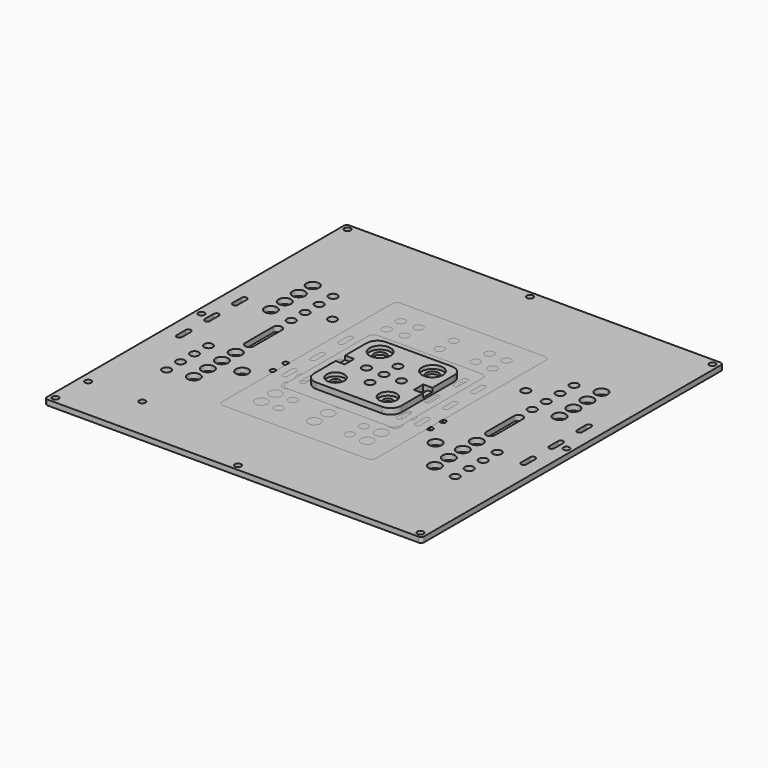
from build123d import *

# Parameters (mm, degrees)
F0_R      = 1.8
F0_R_2    = 2.5
F0_R_3    = 3.6
F0_R_4    = 1.57
F0_R_5    = 1.75
F1_DEPTH  = 3
F2_R      = 3.55
F2_R_2    = 2.55
F3_DEPTH  = 3
F5_R      = 5.05
F5_R_2    = 2.51
F5_R_3    = 6
F6_DEPTH  = 6.35
F5_R_4    = 3.57
F5_R_5    = 2.5
F7_DEPTH  = 4.35
F5_W      = 2.75
F5_H      = 6.7
F8_DEPTH  = 4.17
F9_R      = 3.6
F9_R_2    = 2.5
F10_DEPTH = 3


with BuildPart() as f1:
    # F0 (on Top) → F1 (new body)
    with BuildSketch(Plane.XY):
        with BuildLine():
            Line((106.25, 108), (-106.25, 108))
            ThreePointArc((-106.25, 108), (-107.4874368671, 107.4874368671), (-108, 106.25))
            Line((-108, 106.25), (-108, -106.25))
            ThreePointArc((-108, -106.25), (-107.4874368671, -107.4874368671), (-106.25, -108))
            Line((-106.25, -108), (106.25, -108))
            ThreePointArc((106.25, -108), (107.4874368671, -107.4874368671), (108, -106.25))
            Line((108, -106.25), (108, 106.25))
            ThreePointArc((108, 106.25), (107.4874368671, 107.4874368671), (106.25, 108))
        make_face()
        with Locations((-104.5, -104.5)):
            Circle(F0_R, mode=Mode.SUBTRACT)
        with Locations((-103, -83)):
            Circle(F0_R, mode=Mode.SUBTRACT)
        with Locations((-72, -83)):
            Circle(F0_R, mode=Mode.SUBTRACT)
        with Locations((-82.65, -52.3)):
            Circle(F0_R_2, mode=Mode.SUBTRACT)
        with Locations((-82.65, -42.3)):
            Circle(F0_R_2, mode=Mode.SUBTRACT)
        with Locations((-82.65, -32.3)):
            Circle(F0_R_2, mode=Mode.SUBTRACT)
        with Locations((-69, -49.85)):
            Circle(F0_R_3, mode=Mode.SUBTRACT)
        with Locations((-69, -39.85)):
            Circle(F0_R_3, mode=Mode.SUBTRACT)
        with Locations((-69, -29.85)):
            Circle(F0_R_3, mode=Mode.SUBTRACT)
        with Locations((-55.35, -32.3)):
            Circle(F0_R_3, mode=Mode.SUBTRACT)
        with BuildLine():
            Line((-100.12, -23.25), (-100.12, -16.75))
            ThreePointArc((-100.12, -16.75), (-98.62, -15.25), (-97.12, -16.75))
            Line((-97.12, -16.75), (-97.12, -23.25))
            ThreePointArc((-97.12, -23.25), (-98.62, -24.75), (-100.12, -23.25))
        make_face(mode=Mode.SUBTRACT)
        with Locations((-82.65, -22.3)):
            Circle(F0_R_2, mode=Mode.SUBTRACT)
        with Locations((-69, -19.85)):
            Circle(F0_R_3, mode=Mode.SUBTRACT)
        with Locations((-20.325, -30.32)):
            Circle(F0_R_2, mode=Mode.SUBTRACT)
        with Locations((-45, -23.12)):
            Circle(F0_R_4, mode=Mode.SUBTRACT)
        with Locations((-45, -14)):
            Circle(F0_R_4, mode=Mode.SUBTRACT)
        with Locations((-28, -12.64)):
            Circle(F0_R_5, mode=Mode.SUBTRACT)
        with Locations((-28, -2.5)):
            Circle(F0_R_5, mode=Mode.SUBTRACT)
        with Locations((-10.16, -20.32)):
            Circle(F0_R_2, mode=Mode.SUBTRACT)
        with Locations((-15.17, -12.64)):
            Circle(F0_R_5, mode=Mode.SUBTRACT)
        with Locations((-15.17, -2.5)):
            Circle(F0_R_5, mode=Mode.SUBTRACT)
        with Locations((0, -104.5)):
            Circle(F0_R, mode=Mode.SUBTRACT)
        with Locations((104.5, -104.5)):
            Circle(F0_R, mode=Mode.SUBTRACT)
        with Locations((20.325, -30.32)):
            Circle(F0_R_2, mode=Mode.SUBTRACT)
        with Locations((10.16, -20.32)):
            Circle(F0_R_2, mode=Mode.SUBTRACT)
        with Locations((0, -10)):
            Circle(F0_R_2, mode=Mode.SUBTRACT)
        with Locations((45, -23.12)):
            Circle(F0_R_4, mode=Mode.SUBTRACT)
        with Locations((45, -14)):
            Circle(F0_R_4, mode=Mode.SUBTRACT)
        with Locations((69, -49.85)):
            Circle(F0_R_3, mode=Mode.SUBTRACT)
        with Locations((55.35, -32.3)):
            Circle(F0_R_3, mode=Mode.SUBTRACT)
        with Locations((69, -39.85)):
            Circle(F0_R_3, mode=Mode.SUBTRACT)
        with Locations((69, -29.85)):
            Circle(F0_R_3, mode=Mode.SUBTRACT)
        with Locations((82.65, -52.3)):
            Circle(F0_R_2, mode=Mode.SUBTRACT)
        with Locations((82.65, -42.3)):
            Circle(F0_R_2, mode=Mode.SUBTRACT)
        with Locations((82.65, -32.3)):
            Circle(F0_R_2, mode=Mode.SUBTRACT)
        with Locations((69, -19.85)):
            Circle(F0_R_3, mode=Mode.SUBTRACT)
        with Locations((82.65, -22.3)):
            Circle(F0_R_2, mode=Mode.SUBTRACT)
        with BuildLine():
            Line((97.12, -23.25), (97.12, -16.75))
            ThreePointArc((97.12, -16.75), (98.62, -15.25), (100.12, -16.75))
            Line((100.12, -16.75), (100.12, -23.25))
            ThreePointArc((100.12, -23.25), (98.62, -24.75), (97.12, -23.25))
        make_face(mode=Mode.SUBTRACT)
        with Locations((-104.5, 0)):
            Circle(F0_R, mode=Mode.SUBTRACT)
        with BuildLine():
            ThreePointArc((-100.12, 3.25), (-98.62, 4.75), (-97.12, 3.25))
            Line((-97.12, 3.25), (-97.12, -3.25))
            ThreePointArc((-97.12, -3.25), (-98.62, -4.75), (-100.12, -3.25))
            Line((-100.12, -3.25), (-100.12, 3.25))
        make_face(mode=Mode.SUBTRACT)
        with BuildLine():
            ThreePointArc((-100.12, 23.25), (-98.62, 24.75), (-97.12, 23.25))
            Line((-97.12, 23.25), (-97.12, 16.75))
            ThreePointArc((-97.12, 16.75), (-98.62, 15.25), (-100.12, 16.75))
            Line((-100.12, 16.75), (-100.12, 23.25))
        make_face(mode=Mode.SUBTRACT)
        with Locations((-82.65, 22.3)):
            Circle(F0_R_3, mode=Mode.SUBTRACT)
        with BuildLine():
            Line((-66.5, 10), (-66.5, -10))
            ThreePointArc((-66.5, -10), (-69, -12.5), (-71.5, -10))
            Line((-71.5, -10), (-71.5, 10))
            ThreePointArc((-71.5, 10), (-69, 12.5), (-66.5, 10))
        make_face(mode=Mode.SUBTRACT)
        with Locations((-69, 19.85)):
            Circle(F0_R_2, mode=Mode.SUBTRACT)
        with Locations((-82.65, 32.3)):
            Circle(F0_R_3, mode=Mode.SUBTRACT)
        with Locations((-82.65, 42.3)):
            Circle(F0_R_3, mode=Mode.SUBTRACT)
        with Locations((-82.65, 52.3)):
            Circle(F0_R_3, mode=Mode.SUBTRACT)
        with Locations((-69, 29.85)):
            Circle(F0_R_2, mode=Mode.SUBTRACT)
        with Locations((-69, 39.85)):
            Circle(F0_R_2, mode=Mode.SUBTRACT)
        with Locations((-55.35, 32.3)):
            Circle(F0_R_2, mode=Mode.SUBTRACT)
        with Locations((-69, 49.85)):
            Circle(F0_R_2, mode=Mode.SUBTRACT)
        with Locations((-10.16, 20.32)):
            Circle(F0_R_2, mode=Mode.SUBTRACT)
        with Locations((-20.325, 30.32)):
            Circle(F0_R_2, mode=Mode.SUBTRACT)
        with Locations((-104.5, 104.5)):
            Circle(F0_R, mode=Mode.SUBTRACT)
        Circle(F0_R, mode=Mode.SUBTRACT)
        with Locations((0, 10)):
            Circle(F0_R_2, mode=Mode.SUBTRACT)
        with Locations((10.16, 20.32)):
            Circle(F0_R_2, mode=Mode.SUBTRACT)
        with Locations((20.325, 30.32)):
            Circle(F0_R_2, mode=Mode.SUBTRACT)
        with BuildLine():
            ThreePointArc((71.5, -10), (69, -12.5), (66.5, -10))
            Line((66.5, -10), (66.5, 10))
            ThreePointArc((66.5, 10), (69, 12.5), (71.5, 10))
            Line((71.5, 10), (71.5, -10))
        make_face(mode=Mode.SUBTRACT)
        with Locations((69, 19.85)):
            Circle(F0_R_2, mode=Mode.SUBTRACT)
        with BuildLine():
            ThreePointArc((100.12, -3.25), (98.62, -4.75), (97.12, -3.25))
            Line((97.12, -3.25), (97.12, 3.25))
            ThreePointArc((97.12, 3.25), (98.62, 4.75), (100.12, 3.25))
            Line((100.12, 3.25), (100.12, -3.25))
        make_face(mode=Mode.SUBTRACT)
        with Locations((104.5, 0)):
            Circle(F0_R, mode=Mode.SUBTRACT)
        with Locations((82.65, 22.3)):
            Circle(F0_R_3, mode=Mode.SUBTRACT)
        with BuildLine():
            Line((97.12, 16.75), (97.12, 23.25))
            ThreePointArc((97.12, 23.25), (98.62, 24.75), (100.12, 23.25))
            Line((100.12, 23.25), (100.12, 16.75))
            ThreePointArc((100.12, 16.75), (98.62, 15.25), (97.12, 16.75))
        make_face(mode=Mode.SUBTRACT)
        with Locations((55.35, 32.3)):
            Circle(F0_R_2, mode=Mode.SUBTRACT)
        with Locations((69, 29.85)):
            Circle(F0_R_2, mode=Mode.SUBTRACT)
        with Locations((69, 39.85)):
            Circle(F0_R_2, mode=Mode.SUBTRACT)
        with Locations((69, 49.85)):
            Circle(F0_R_2, mode=Mode.SUBTRACT)
        with Locations((82.65, 32.3)):
            Circle(F0_R_3, mode=Mode.SUBTRACT)
        with Locations((82.65, 42.3)):
            Circle(F0_R_3, mode=Mode.SUBTRACT)
        with Locations((82.65, 52.3)):
            Circle(F0_R_3, mode=Mode.SUBTRACT)
        with Locations((0, 104.5)):
            Circle(F0_R, mode=Mode.SUBTRACT)
        with Locations((104.5, 104.5)):
            Circle(F0_R, mode=Mode.SUBTRACT)
    extrude(amount=F1_DEPTH)


with BuildPart() as f3:
    # F2 (on Top) → F3 (new body)
    with BuildSketch(Plane.XY):
        with BuildLine():
            Line((41, 63.5), (-41, 63.5))
            ThreePointArc((-41, 63.5), (-43.1213203436, 62.6213203436), (-44, 60.5))
            Line((-44, 60.5), (-44, -60.5))
            ThreePointArc((-44, -60.5), (-43.1213203436, -62.6213203436), (-41, -63.5))
            Line((-41, -63.5), (41, -63.5))
            ThreePointArc((41, -63.5), (43.1213203436, -62.6213203436), (44, -60.5))
            Line((44, -60.5), (44, 60.5))
            ThreePointArc((44, 60.5), (43.1213203436, 62.6213203436), (41, 63.5))
        make_face()
        with Locations((-30.32, -49.85)):
            Circle(F2_R, mode=Mode.SUBTRACT)
        with Locations((-30.32, -39.85)):
            Circle(F2_R, mode=Mode.SUBTRACT)
        with Locations((-20.32, -49.85)):
            Circle(F2_R_2, mode=Mode.SUBTRACT)
        with Locations((-20.32, -39.85)):
            Circle(F2_R_2, mode=Mode.SUBTRACT)
        with BuildLine():
            ThreePointArc((-39.5, -16.75), (-38, -15.25), (-36.5, -16.75))
            Line((-36.5, -16.75), (-36.5, -23.25))
            ThreePointArc((-36.5, -23.25), (-38, -24.75), (-39.5, -23.25))
            Line((-39.5, -23.25), (-39.5, -16.75))
        make_face(mode=Mode.SUBTRACT)
        with Locations((-30.32, -29.85)):
            Circle(F2_R, mode=Mode.SUBTRACT)
        with Locations((-30.32, -19.85)):
            Circle(F2_R, mode=Mode.SUBTRACT)
        with Locations((-20.32, -29.85)):
            Circle(F2_R_2, mode=Mode.SUBTRACT)
        with Locations((-20.32, -19.85)):
            Circle(F2_R_2, mode=Mode.SUBTRACT)
        with Locations((-10, -30.32)):
            Circle(F2_R_2, mode=Mode.SUBTRACT)
        with Locations((-10, -20.32)):
            Circle(F2_R_2, mode=Mode.SUBTRACT)
        with Locations((-20.32, -9.85)):
            Circle(F2_R_2, mode=Mode.SUBTRACT)
        with Locations((-14.825, -14.825)):
            Circle(F2_R_2, mode=Mode.SUBTRACT)
        with Locations((0, -49.85)):
            Circle(F2_R, mode=Mode.SUBTRACT)
        with Locations((20.32, -49.85)):
            Circle(F2_R_2, mode=Mode.SUBTRACT)
        with Locations((0, -39.85)):
            Circle(F2_R, mode=Mode.SUBTRACT)
        with Locations((20.32, -39.85)):
            Circle(F2_R_2, mode=Mode.SUBTRACT)
        with Locations((30.32, -49.85)):
            Circle(F2_R, mode=Mode.SUBTRACT)
        with Locations((30.32, -39.85)):
            Circle(F2_R, mode=Mode.SUBTRACT)
        with Locations((0, -29.85)):
            Circle(F2_R, mode=Mode.SUBTRACT)
        with Locations((10, -30.32)):
            Circle(F2_R_2, mode=Mode.SUBTRACT)
        with Locations((0, -19.85)):
            Circle(F2_R, mode=Mode.SUBTRACT)
        with Locations((10, -20.32)):
            Circle(F2_R_2, mode=Mode.SUBTRACT)
        with Locations((20.32, -29.85)):
            Circle(F2_R_2, mode=Mode.SUBTRACT)
        with Locations((20.32, -19.85)):
            Circle(F2_R_2, mode=Mode.SUBTRACT)
        with Locations((0, -10)):
            Circle(F2_R_2, mode=Mode.SUBTRACT)
        with Locations((14.825, -14.825)):
            Circle(F2_R_2, mode=Mode.SUBTRACT)
        with Locations((20.32, -9.85)):
            Circle(F2_R_2, mode=Mode.SUBTRACT)
        with Locations((30.32, -29.85)):
            Circle(F2_R, mode=Mode.SUBTRACT)
        with Locations((30.32, -19.85)):
            Circle(F2_R, mode=Mode.SUBTRACT)
        with BuildLine():
            Line((36.5, -23.25), (36.5, -16.75))
            ThreePointArc((36.5, -16.75), (38, -15.25), (39.5, -16.75))
            Line((39.5, -16.75), (39.5, -23.25))
            ThreePointArc((39.5, -23.25), (38, -24.75), (36.5, -23.25))
        make_face(mode=Mode.SUBTRACT)
        with BuildLine():
            Line((-39.5, -3.25), (-39.5, 3.25))
            ThreePointArc((-39.5, 3.25), (-38, 4.75), (-36.5, 3.25))
            Line((-36.5, 3.25), (-36.5, -3.25))
            ThreePointArc((-36.5, -3.25), (-38, -4.75), (-39.5, -3.25))
        make_face(mode=Mode.SUBTRACT)
        with BuildLine():
            Line((-27.82, 10), (-27.82, -10))
            ThreePointArc((-27.82, -10), (-30.32, -12.5), (-32.82, -10))
            Line((-32.82, -10), (-32.82, 10))
            ThreePointArc((-32.82, 10), (-30.32, 12.5), (-27.82, 10))
        make_face(mode=Mode.SUBTRACT)
        with BuildLine():
            Line((-36.5, 23.25), (-36.5, 16.75))
            ThreePointArc((-36.5, 16.75), (-38, 15.25), (-39.5, 16.75))
            Line((-39.5, 16.75), (-39.5, 23.25))
            ThreePointArc((-39.5, 23.25), (-38, 24.75), (-36.5, 23.25))
        make_face(mode=Mode.SUBTRACT)
        with Locations((-30.32, 19.85)):
            Circle(F2_R_2, mode=Mode.SUBTRACT)
        with Locations((-30.32, 29.85)):
            Circle(F2_R_2, mode=Mode.SUBTRACT)
        with Locations((-20.32, 0.15)):
            Circle(F2_R_2, mode=Mode.SUBTRACT)
        with Locations((-20.32, 10.15)):
            Circle(F2_R_2, mode=Mode.SUBTRACT)
        with Locations((-14.825, 14.825)):
            Circle(F2_R_2, mode=Mode.SUBTRACT)
        with Locations((-10, 0)):
            Circle(F2_R_2, mode=Mode.SUBTRACT)
        with Locations((-20.32, 20.15)):
            Circle(F2_R_2, mode=Mode.SUBTRACT)
        with Locations((-20.32, 30.15)):
            Circle(F2_R_2, mode=Mode.SUBTRACT)
        with Locations((-10, 20.32)):
            Circle(F2_R_2, mode=Mode.SUBTRACT)
        with Locations((-10, 30.32)):
            Circle(F2_R_2, mode=Mode.SUBTRACT)
        with Locations((-30.32, 39.85)):
            Circle(F2_R_2, mode=Mode.SUBTRACT)
        with Locations((-30.32, 49.85)):
            Circle(F2_R_2, mode=Mode.SUBTRACT)
        with Locations((-20.32, 40.15)):
            Circle(F2_R_2, mode=Mode.SUBTRACT)
        with Locations((-20.32, 50.15)):
            Circle(F2_R_2, mode=Mode.SUBTRACT)
        Circle(F2_R_2, mode=Mode.SUBTRACT)
        with Locations((10, 0)):
            Circle(F2_R_2, mode=Mode.SUBTRACT)
        with Locations((0, 10)):
            Circle(F2_R_2, mode=Mode.SUBTRACT)
        with Locations((20.32, 0.15)):
            Circle(F2_R_2, mode=Mode.SUBTRACT)
        with Locations((14.825, 14.825)):
            Circle(F2_R_2, mode=Mode.SUBTRACT)
        with Locations((20.32, 10.15)):
            Circle(F2_R_2, mode=Mode.SUBTRACT)
        with Locations((0, 19.85)):
            Circle(F2_R_2, mode=Mode.SUBTRACT)
        with Locations((10, 20.32)):
            Circle(F2_R_2, mode=Mode.SUBTRACT)
        with Locations((0, 29.85)):
            Circle(F2_R_2, mode=Mode.SUBTRACT)
        with Locations((10, 30.32)):
            Circle(F2_R_2, mode=Mode.SUBTRACT)
        with Locations((20.32, 20.15)):
            Circle(F2_R_2, mode=Mode.SUBTRACT)
        with Locations((20.32, 30.15)):
            Circle(F2_R_2, mode=Mode.SUBTRACT)
        with BuildLine():
            Line((32.82, 10), (32.82, -10))
            ThreePointArc((32.82, -10), (30.32, -12.5), (27.82, -10))
            Line((27.82, -10), (27.82, 10))
            ThreePointArc((27.82, 10), (30.32, 12.5), (32.82, 10))
        make_face(mode=Mode.SUBTRACT)
        with BuildLine():
            ThreePointArc((36.5, 3.25), (38, 4.75), (39.5, 3.25))
            Line((39.5, 3.25), (39.5, -3.25))
            ThreePointArc((39.5, -3.25), (38, -4.75), (36.5, -3.25))
            Line((36.5, -3.25), (36.5, 3.25))
        make_face(mode=Mode.SUBTRACT)
        with Locations((30.32, 19.85)):
            Circle(F2_R_2, mode=Mode.SUBTRACT)
        with Locations((30.32, 29.85)):
            Circle(F2_R_2, mode=Mode.SUBTRACT)
        with BuildLine():
            ThreePointArc((36.5, 23.25), (38, 24.75), (39.5, 23.25))
            Line((39.5, 23.25), (39.5, 16.75))
            ThreePointArc((39.5, 16.75), (38, 15.25), (36.5, 16.75))
            Line((36.5, 16.75), (36.5, 23.25))
        make_face(mode=Mode.SUBTRACT)
        with Locations((0, 39.85)):
            Circle(F2_R_2, mode=Mode.SUBTRACT)
        with Locations((20.32, 40.15)):
            Circle(F2_R_2, mode=Mode.SUBTRACT)
        with Locations((0, 49.85)):
            Circle(F2_R_2, mode=Mode.SUBTRACT)
        with Locations((20.32, 50.15)):
            Circle(F2_R_2, mode=Mode.SUBTRACT)
        with Locations((30.32, 39.85)):
            Circle(F2_R_2, mode=Mode.SUBTRACT)
        with Locations((30.32, 49.85)):
            Circle(F2_R_2, mode=Mode.SUBTRACT)
    extrude(amount=F3_DEPTH)


with BuildPart() as f6:
    # F5 (on Top) → F6 (new body)
    with BuildSketch(Plane.XY):
        with BuildLine():
            Line((-18.83, -25), (18.83, -25))
            ThreePointArc((18.83, -25), (23.1928488399, -23.1928488399), (25, -18.83))
            Line((25, -18.83), (25, -3.35))
            Line((25, -3.35), (22.25, -3.35))
            Line((22.25, -3.35), (19.75, -3.35))
            Line((19.75, -3.35), (19.75, 3.35))
            Line((19.75, 3.35), (22.25, 3.35))
            Line((22.25, 3.35), (25, 3.35))
            Line((25, 3.35), (25, 18.83))
            ThreePointArc((25, 18.83), (23.1928488399, 23.1928488399), (18.83, 25))
            Line((18.83, 25), (-18.83, 25))
            ThreePointArc((-18.83, 25), (-23.1928488399, 23.1928488399), (-25, 18.83))
            Line((-25, 18.83), (-25, 3.35))
            Line((-25, 3.35), (-22.25, 3.35))
            Line((-22.25, 3.35), (-19.75, 3.35))
            Line((-19.75, 3.35), (-19.75, -3.35))
            Line((-19.75, -3.35), (-22.25, -3.35))
            Line((-22.25, -3.35), (-25, -3.35))
            Line((-25, -3.35), (-25, -18.83))
            ThreePointArc((-25, -18.83), (-23.1928488399, -23.1928488399), (-18.83, -25))
        make_face()
        with Locations((-15, -15.95)):
            Circle(F5_R, mode=Mode.SUBTRACT)
        with Locations((0, -10)):
            Circle(F5_R_2, mode=Mode.SUBTRACT)
        with Locations((15, -15.95)):
            Circle(F5_R, mode=Mode.SUBTRACT)
        with Locations((-10, 0)):
            Circle(F5_R_2, mode=Mode.SUBTRACT)
        Circle(F5_R_2, mode=Mode.SUBTRACT)
        with Locations((0, 10)):
            Circle(F5_R_2, mode=Mode.SUBTRACT)
        with Locations((-15, 15.95)):
            Circle(F5_R_3, mode=Mode.SUBTRACT)
        with Locations((10, 0)):
            Circle(F5_R_2, mode=Mode.SUBTRACT)
        with Locations((15, 15.95)):
            Circle(F5_R_3, mode=Mode.SUBTRACT)
    extrude(amount=F6_DEPTH)

    # F5 (on Top) → F7 (join)
    with BuildSketch(Plane.XY):
        with Locations((-15, 15.95)):
            Circle(F5_R_3)
        with Locations((-15, 15.95)):
            Circle(F5_R_4, mode=Mode.SUBTRACT)
        with Locations((15, 15.95)):
            Circle(F5_R_3)
        with Locations((15, 15.95)):
            Circle(F5_R_4, mode=Mode.SUBTRACT)
        with Locations((15, -15.95)):
            Circle(F5_R)
        with Locations((15, -15.95)):
            Circle(F5_R_5, mode=Mode.SUBTRACT)
        with Locations((-15, -15.95)):
            Circle(F5_R)
        with Locations((-15, -15.95)):
            Circle(F5_R_5, mode=Mode.SUBTRACT)
    extrude(amount=F7_DEPTH)

    # F5 (on Top) → F8 (join)
    with BuildSketch(Plane.XY):
        with Locations((-23.625, 0)):
            Rectangle(F5_W, F5_H)
        with Locations((23.625, 0)):
            Rectangle(F5_W, F5_H)
    extrude(amount=F8_DEPTH)


with BuildPart() as f10:
    # F9 (on Top) → F10 (new body)
    with BuildSketch(Plane.XY):
        with BuildLine():
            ThreePointArc((-32.75, -29.37), (-31.7600209204, -31.7600209204), (-29.37, -32.75))
            Line((-29.37, -32.75), (29.37, -32.75))
            ThreePointArc((29.37, -32.75), (31.7600209204, -31.7600209204), (32.75, -29.37))
            Line((32.75, -29.37), (32.75, 29.37))
            ThreePointArc((32.75, 29.37), (31.7600209204, 31.7600209204), (29.37, 32.75))
            Line((29.37, 32.75), (-29.37, 32.75))
            ThreePointArc((-29.37, 32.75), (-31.7600209204, 31.7600209204), (-32.75, 29.37))
            Line((-32.75, 29.37), (-32.75, -29.37))
        make_face()
        with BuildLine():
            Line((-26.2, -16.895), (-26.2, -23.395))
            ThreePointArc((-26.2, -23.395), (-27.7, -24.895), (-29.2, -23.395))
            Line((-29.2, -23.395), (-29.2, -16.895))
            ThreePointArc((-29.2, -16.895), (-27.7, -15.395), (-26.2, -16.895))
        make_face(mode=Mode.SUBTRACT)
        with Locations((-20, -19.85)):
            Circle(F9_R, mode=Mode.SUBTRACT)
        with Locations((-10, -19.85)):
            Circle(F9_R_2, mode=Mode.SUBTRACT)
        with Locations((0, -19.85)):
            Circle(F9_R, mode=Mode.SUBTRACT)
        with Locations((10, -19.85)):
            Circle(F9_R_2, mode=Mode.SUBTRACT)
        with Locations((20, -19.85)):
            Circle(F9_R, mode=Mode.SUBTRACT)
        with BuildLine():
            Line((29.2, -16.895), (29.2, -23.395))
            ThreePointArc((29.2, -23.395), (27.7, -24.895), (26.2, -23.395))
            Line((26.2, -23.395), (26.2, -16.895))
            ThreePointArc((26.2, -16.895), (27.7, -15.395), (29.2, -16.895))
        make_face(mode=Mode.SUBTRACT)
        with Locations((0, -10)):
            Circle(F9_R_2, mode=Mode.SUBTRACT)
        with BuildLine():
            Line((-26.2, 3.25), (-26.2, -3.25))
            ThreePointArc((-26.2, -3.25), (-27.7, -4.75), (-29.2, -3.25))
            Line((-29.2, -3.25), (-29.2, 3.25))
            ThreePointArc((-29.2, 3.25), (-27.7, 4.75), (-26.2, 3.25))
        make_face(mode=Mode.SUBTRACT)
        with BuildLine():
            Line((-22.5, -10.32), (-22.5, 10.32))
            ThreePointArc((-22.5, 10.32), (-20, 12.82), (-17.5, 10.32))
            Line((-17.5, 10.32), (-17.5, -10.32))
            ThreePointArc((-17.5, -10.32), (-20, -12.82), (-22.5, -10.32))
        make_face(mode=Mode.SUBTRACT)
        with Locations((-10, 0)):
            Circle(F9_R_2, mode=Mode.SUBTRACT)
        with BuildLine():
            Line((-29.2, 16.895), (-29.2, 23.395))
            ThreePointArc((-29.2, 23.395), (-27.7, 24.895), (-26.2, 23.395))
            Line((-26.2, 23.395), (-26.2, 16.895))
            ThreePointArc((-26.2, 16.895), (-27.7, 15.395), (-29.2, 16.895))
        make_face(mode=Mode.SUBTRACT)
        with Locations((-20, 19.85)):
            Circle(F9_R_2, mode=Mode.SUBTRACT)
        with Locations((-10, 19.85)):
            Circle(F9_R_2, mode=Mode.SUBTRACT)
        Circle(F9_R_2, mode=Mode.SUBTRACT)
        with Locations((10, 0)):
            Circle(F9_R_2, mode=Mode.SUBTRACT)
        with Locations((0, 10)):
            Circle(F9_R_2, mode=Mode.SUBTRACT)
        with BuildLine():
            ThreePointArc((17.5, 10.32), (20, 12.82), (22.5, 10.32))
            Line((22.5, 10.32), (22.5, -10.32))
            ThreePointArc((22.5, -10.32), (20, -12.82), (17.5, -10.32))
            Line((17.5, -10.32), (17.5, 10.32))
        make_face(mode=Mode.SUBTRACT)
        with BuildLine():
            Line((29.2, 3.25), (29.2, -3.25))
            ThreePointArc((29.2, -3.25), (27.7, -4.75), (26.2, -3.25))
            Line((26.2, -3.25), (26.2, 3.25))
            ThreePointArc((26.2, 3.25), (27.7, 4.75), (29.2, 3.25))
        make_face(mode=Mode.SUBTRACT)
        with Locations((0, 19.85)):
            Circle(F9_R_2, mode=Mode.SUBTRACT)
        with Locations((10, 19.85)):
            Circle(F9_R_2, mode=Mode.SUBTRACT)
        with Locations((20, 19.85)):
            Circle(F9_R_2, mode=Mode.SUBTRACT)
        with BuildLine():
            Line((29.2, 23.395), (29.2, 16.895))
            ThreePointArc((29.2, 16.895), (27.7, 15.395), (26.2, 16.895))
            Line((26.2, 16.895), (26.2, 23.395))
            ThreePointArc((26.2, 23.395), (27.7, 24.895), (29.2, 23.395))
        make_face(mode=Mode.SUBTRACT)
    extrude(amount=F10_DEPTH)


solid = Compound([f1.part, f3.part, f6.part, f10.part])
